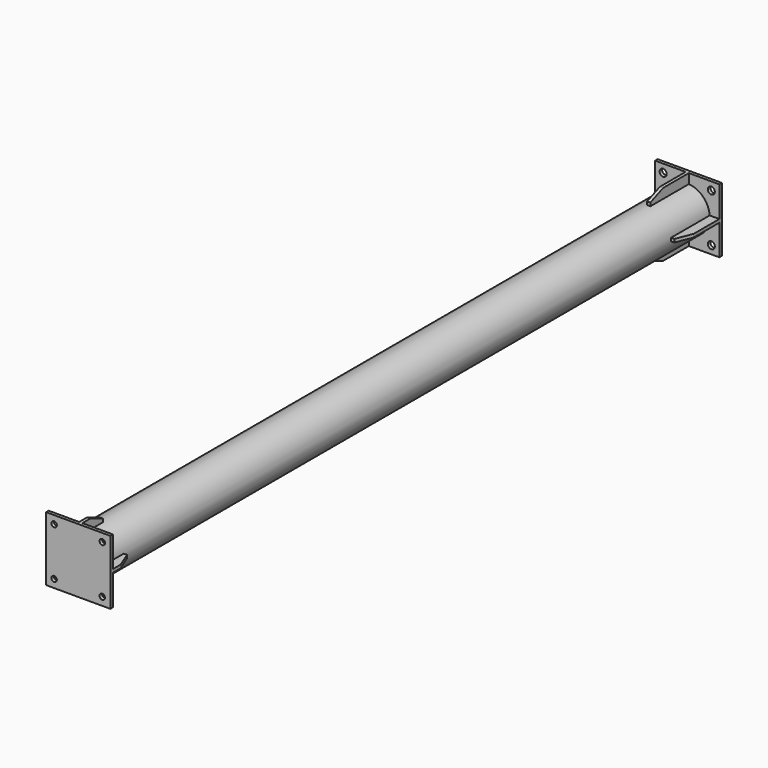
from build123d import *

# Parameters (mm, degrees)
F0_R          = 70
F0_R_2        = 65
F1_DEPTH      = 2360
F2_W          = 200
F2_H          = 200
F2_R          = 11
F3_DEPTH      = 10
F4_W          = 30.1787997812
F4_H          = 10
F4_W_2        = 10
F4_H_2        = 30.1787997812
F5_DEPTH      = 150
F6_T1_DEPTH   = 269.311363913
F6_T3_DEPTH   = 269.311363913
F6_T8_DEPTH   = 269.311363913
F6_S9_R       = 70
F6_T10_DEPTH  = 139
F8_W          = 200
F8_H          = 200
F8_R          = 8.5
F9_DEPTH      = 10
F10_W         = 10
F10_H         = 30.1787997812
F10_W_2       = 30.1787997812
F10_H_2       = 10
F11_DEPTH     = 80
F12_T1_DEPTH  = 269.311363913
F12_T3_DEPTH  = 269.311363913
F12_T8_DEPTH  = 269.311363913
F12_S9_R      = 70
F12_T10_DEPTH = 139
F12_T14_DEPTH = 269.311363913
F12_S15_R     = 70
F12_T16_DEPTH = 139


# Not quite as in the source:
# - a fillet or chamfer that OpenCascade refuses, or shapes differently, is made with other operations: its cross-section is extruded or revolved along the edge and cut away or added


with BuildPart() as f1:
    # F0 (on Front) → F1 (new body)
    with BuildSketch(Plane.XZ):
        Circle(F0_R)
        Circle(F0_R_2, mode=Mode.SUBTRACT)
    extrude(amount=F1_DEPTH)

    # F2 (on Front) → F3 (join)
    with BuildSketch(Plane.XZ):
        Rectangle(F2_W, F2_H)
        with Locations((-75, -75)):
            Circle(F2_R, mode=Mode.SUBTRACT)
        with Locations((75, -75)):
            Circle(F2_R, mode=Mode.SUBTRACT)
        with Locations((-75, 75)):
            Circle(F2_R, mode=Mode.SUBTRACT)
        with Locations((75, 75)):
            Circle(F2_R, mode=Mode.SUBTRACT)
    extrude(amount=-F3_DEPTH)

    # F4 (on Front) → F5 (join)
    with BuildSketch(Plane.XZ):
        with Locations((-84.9106001094, 0)):
            Rectangle(F4_W, F4_H)
        with Locations((0, 84.9106001094)):
            Rectangle(F4_W_2, F4_H_2)
        with Locations((84.9106001094, 0)):
            Rectangle(F4_W, F4_H)
        with Locations((0, -84.9106001094)):
            Rectangle(F4_W_2, F4_H_2)
    extrude(amount=F5_DEPTH)

    # F6: chamfer of 50 x 20 on 4 edges, made by hand

    # F6_s2 → F6_t1 (cut)
    with BuildSketch(Plane.YZ.offset(-134.6556819565)):
        Polygon((-100, 100), (-150, 80), (-150, 100), align=None)
        Polygon((-100, -100), (-150, -80), (-150, -100), align=None)
    extrude(amount=F6_T1_DEPTH, mode=Mode.SUBTRACT)

    # F6_s4 → F6_t3 (cut)
    with BuildSketch(Plane.XY.offset(-134.6556819565)):
        Polygon((100, -100), (80, -150), (100, -150), align=None)
    extrude(amount=F6_T3_DEPTH, mode=Mode.SUBTRACT)


with BuildPart() as f6_tool6:
    # F6_s7 → F6_t8 (new body)
    with BuildSketch(Plane.XY.offset(134.6556819565)):
        Polygon((-100, -130), (-50, -150), (-100, -150), align=None)
    extrude(amount=-F6_T8_DEPTH)

    # F6_s9 → F6_t10 (cut, symmetric)
    with BuildSketch(Plane.XZ.offset(140)):
        Circle(F6_S9_R)
    extrude(amount=F6_T10_DEPTH, both=True, mode=Mode.SUBTRACT)


with BuildPart() as f1_1:
    add(f1.part)

    # F6_t5: cut F6_tool6
    add(f6_tool6.part, mode=Mode.SUBTRACT)

    # F8 (on offset) → F9 (join)
    with BuildSketch(Plane.XZ.offset(2360)):
        Rectangle(F8_W, F8_H)
        with Locations((-75, -75)):
            Circle(F8_R, mode=Mode.SUBTRACT)
        with Locations((75, -75)):
            Circle(F8_R, mode=Mode.SUBTRACT)
        with Locations((-75, 75)):
            Circle(F8_R, mode=Mode.SUBTRACT)
        with Locations((75, 75)):
            Circle(F8_R, mode=Mode.SUBTRACT)
    extrude(amount=F9_DEPTH)

    # F10 (on face) → F11 (join)
    with BuildSketch(Plane(origin=(0, -2360, 0), x_dir=(-1, 0, 0), z_dir=(0, 1, 0))):
        with Locations((0, 84.9106001094)):
            Rectangle(F10_W, F10_H)
        with Locations((84.9106001094, 0)):
            Rectangle(F10_W_2, F10_H_2)
        with Locations((0, -84.9106001094)):
            Rectangle(F10_W, F10_H)
        with Locations((-84.9106001094, 0)):
            Rectangle(F10_W_2, F10_H_2)
    extrude(amount=F11_DEPTH)

    # F12: chamfer of 20 x 50 on 4 edges, made by hand

    # F12_s2 → F12_t1 (cut)
    with BuildSketch(Plane.YZ.offset(-134.6556819565)):
        Polygon((-2330, 100), (-2280, 80), (-2280, 100), align=None)
    extrude(amount=F12_T1_DEPTH, mode=Mode.SUBTRACT)

    # F12_s4 → F12_t3 (cut)
    with BuildSketch(Plane.XY.offset(-134.6556819565)):
        Polygon((100, -2330), (80, -2280), (100, -2280), align=None)
    extrude(amount=F12_T3_DEPTH, mode=Mode.SUBTRACT)


with BuildPart() as f12_tool6:
    # F12_s7 → F12_t8 (new body)
    with BuildSketch(Plane.XY.offset(-134.6556819565)):
        Polygon((-100, -2300), (-50, -2280), (-100, -2280), align=None)
    extrude(amount=F12_T8_DEPTH)

    # F12_s9 → F12_t10 (cut, symmetric)
    with BuildSketch(Plane.XZ.offset(2290)):
        Circle(F12_S9_R)
    extrude(amount=F12_T10_DEPTH, both=True, mode=Mode.SUBTRACT)


with BuildPart() as f1_2:
    add(f1_1.part)

    # F12_t5: cut F12_tool6
    add(f12_tool6.part, mode=Mode.SUBTRACT)


with BuildPart() as f12_tool12:
    # F12_s13 → F12_t14 (new body)
    with BuildSketch(Plane.YZ.offset(134.6556819565)):
        Polygon((-2300, -100), (-2280, -50), (-2280, -100), align=None)
    extrude(amount=-F12_T14_DEPTH)

    # F12_s15 → F12_t16 (cut, symmetric)
    with BuildSketch(Plane.XZ.offset(2290)):
        Circle(F12_S15_R)
    extrude(amount=F12_T16_DEPTH, both=True, mode=Mode.SUBTRACT)


with BuildPart() as f1_3:
    add(f1_2.part)

    # F12_t11: cut F12_tool12
    add(f12_tool12.part, mode=Mode.SUBTRACT)


solid = f1_3.part
